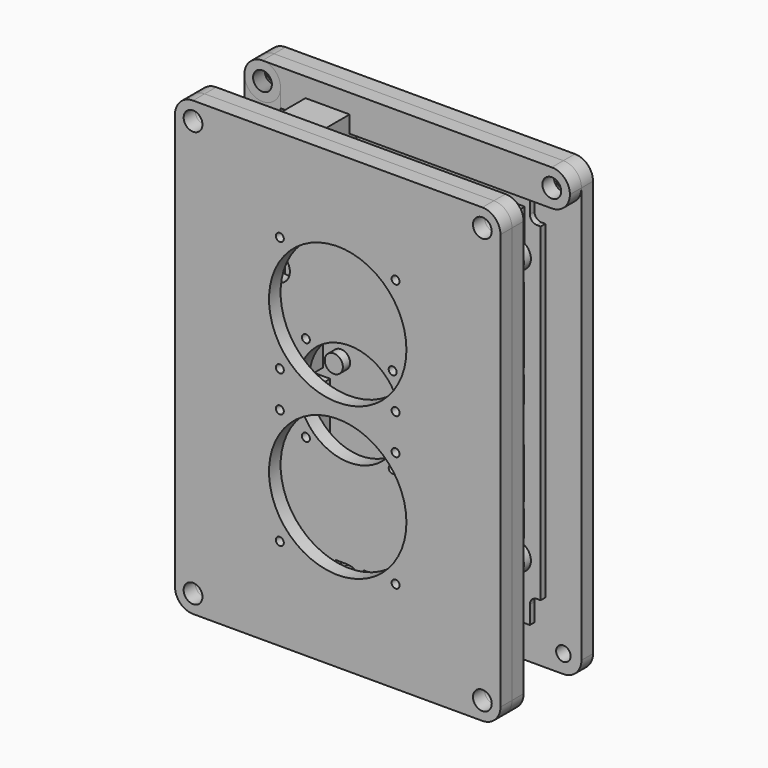
from build123d import *

# Parameters (mm, degrees)
F0_R            = 2
F0_R_2          = 1.5
F0_R_3          = 2.6
F1_DEPTH        = 4
F2_R            = 2.1
F3_DEPTH        = 4
F4_R            = 2.6
F5_DEPTH        = 4
F7_DEPTH        = 4
F8_R            = 2
F9_DEPTH        = 1.6
F10_W           = 12.2
F10_H           = 4.7
F10_H_2         = 11.8
F11_DEPTH       = 10.8
F10_W_2         = 10
F10_H_3         = 9.1
F12_DEPTH       = 12.5
F10_W_3         = 32
F10_H_4         = 7
F13_DEPTH       = 8.85
F14_SIZE2       = 4
F14_SIZE        = 1.5
F15_SIZE2       = 5
F15_SIZE        = 2
F10_W_4         = 7
F10_H_5         = 21
F16_DEPTH       = 8.8
F10_W_5         = 52.5
F10_H_6         = 9.6
F17_DEPTH       = 12.7
F10_H_7         = 14
F18_DEPTH       = 8.8
F19_SIZE2       = 4
F19_SIZE        = 1.5
F10_W_6         = 5
F10_H_8         = 7.25
F20_DEPTH       = 8.6
F21_SIZE2       = 1.5
F21_SIZE        = 4
F21_2_SIZE2     = 1.5
F21_2_SIZE      = 4
F21_3_SIZE2     = 1.5
F21_3_SIZE      = 4
F21_4_SIZE2     = 1.5
F21_4_SIZE      = 4
F21_5_SIZE2     = 1.5
F21_5_SIZE      = 4
F21_6_SIZE2     = 1.5
F21_6_SIZE      = 4
F10_R           = 2.5
F22_DEPTH       = 2.5
F23_R           = 2.6
F24_DEPTH       = 4
F26_R           = 2.6
F26_R_2         = 3.75
F27_DEPTH       = 4
F28_TEXT_SIZE   = 11.6510510219
F28_TEXT_SIZE_2 = 9.4254123618
F29_DEPTH       = 2
F30_R           = 1.1
F30_R_2         = 14.25
F31_DEPTH       = 25
F34_R           = 2.6
F34_R_2         = 1.1
F34_R_3         = 19
F35_DEPTH       = 4


# Not quite as in the source:
# - Text() gives the source's letters only with a copy of the font that has no kerning and outlines rounded to 1/6400 em; it was checked with that copy


with BuildPart() as f1:
    # F0 (on Front) → F1 (new body)
    with BuildSketch(Plane.XZ):
        with BuildLine():
            Line((-40, -62.5), (40, -62.5))
            ThreePointArc((40, -62.5), (43.5355339059, -61.0355339059), (45, -57.5))
            Line((45, -57.5), (45, 57.5))
            ThreePointArc((45, 57.5), (43.5355339059, 61.0355339059), (40, 62.5))
            Line((40, 62.5), (-40, 62.5))
            ThreePointArc((-40, 62.5), (-43.5355339059, 61.0355339059), (-45, 57.5))
            Line((-45, 57.5), (-45, -57.5))
            ThreePointArc((-45, -57.5), (-43.5355339059, -61.0355339059), (-40, -62.5))
        make_face()
        with Locations((-40, -57.5)):
            Circle(F0_R, mode=Mode.SUBTRACT)
        with Locations((-28.55, -36.75)):
            Circle(F0_R_2, mode=Mode.SUBTRACT)
        with Locations((-10, -20)):
            Circle(F0_R_3, mode=Mode.SUBTRACT)
        with Locations((40, -57.5)):
            Circle(F0_R, mode=Mode.SUBTRACT)
        with Locations((28.55, -36.75)):
            Circle(F0_R_2, mode=Mode.SUBTRACT)
        with Locations((10, -20)):
            Circle(F0_R_3, mode=Mode.SUBTRACT)
        with Locations((-10, 20)):
            Circle(F0_R_3, mode=Mode.SUBTRACT)
        with Locations((-28.55, 36.75)):
            Circle(F0_R_2, mode=Mode.SUBTRACT)
        with Locations((-40, 57.5)):
            Circle(F0_R, mode=Mode.SUBTRACT)
        with Locations((10, 20)):
            Circle(F0_R_3, mode=Mode.SUBTRACT)
        with Locations((28.55, 36.75)):
            Circle(F0_R_2, mode=Mode.SUBTRACT)
        with Locations((40, 57.5)):
            Circle(F0_R, mode=Mode.SUBTRACT)
    extrude(amount=F1_DEPTH)


with BuildPart() as f3:
    # F2 (on face) → F3 (new body)
    with BuildSketch(Plane.XZ.offset(4)):
        with BuildLine():
            ThreePointArc((-28.55, 40.5), (-32.3, 36.75), (-28.55, 33))
            Line((-28.55, 33), (28.55, 33))
            ThreePointArc((28.55, 33), (32.3, 36.75), (28.55, 40.5))
            Line((28.55, 40.5), (-28.55, 40.5))
        make_face()
        with Locations((-28.55, 36.75)):
            Circle(F2_R, mode=Mode.SUBTRACT)
        with BuildLine():
            ThreePointArc((30.65, 36.75), (28.55, 34.65), (26.45, 36.75))
            ThreePointArc((26.45, 36.75), (28.55, 38.85), (30.65, 36.75))
        make_face(mode=Mode.SUBTRACT)
    extrude(amount=F3_DEPTH)


with BuildPart() as f3b:
    # F2 (on face) → F3, piece 2 (new body)
    with BuildSketch(Plane.XZ.offset(4)):
        with BuildLine():
            ThreePointArc((-28.55, -33), (-32.3, -36.75), (-28.55, -40.5))
            Line((-28.55, -40.5), (28.55, -40.5))
            ThreePointArc((28.55, -40.5), (32.3, -36.75), (28.55, -33))
            Line((28.55, -33), (-28.55, -33))
        make_face()
        with Locations((-28.55, -36.75)):
            Circle(F2_R, mode=Mode.SUBTRACT)
        with BuildLine():
            ThreePointArc((30.65, -36.75), (28.55, -38.85), (26.45, -36.75))
            ThreePointArc((26.45, -36.75), (28.55, -34.65), (30.65, -36.75))
        make_face(mode=Mode.SUBTRACT)
    extrude(amount=F3_DEPTH)


with BuildPart() as f5:
    # F4 (on face) → F5 (new body)
    with BuildSketch(Plane.XZ.offset(4)):
        with BuildLine():
            ThreePointArc((-45, 57.5), (-43.5355339059, 53.9644660941), (-40, 52.5))
            Line((-40, 52.5), (40, 52.5))
            ThreePointArc((40, 52.5), (43.5355339059, 53.9644660941), (45, 57.5))
            ThreePointArc((45, 57.5), (43.5355339059, 61.0355339059), (40, 62.5))
            Line((40, 62.5), (-40, 62.5))
            ThreePointArc((-40, 62.5), (-43.5355339059, 61.0355339059), (-45, 57.5))
        make_face()
        with Locations((-40, 57.5)):
            Circle(F4_R, mode=Mode.SUBTRACT)
        with BuildLine():
            ThreePointArc((42.6, 57.5), (40, 54.9), (37.4, 57.5))
            ThreePointArc((37.4, 57.5), (40, 60.1), (42.6, 57.5))
        make_face(mode=Mode.SUBTRACT)
    extrude(amount=F5_DEPTH)


with BuildPart() as f7:
    # F6 (on face) → F7 (new body)
    with BuildSketch(Plane.XZ.offset(4)):
        with BuildLine():
            ThreePointArc((-40, 62.5), (-43.5355339059, 61.0355339059), (-45, 57.5))
            Line((-45, 57.5), (-45, -57.5))
            ThreePointArc((-45, -57.5), (-43.5355339059, -61.0355339059), (-40, -62.5))
            ThreePointArc((-40, -62.5), (-36.4644660941, -61.0355339059), (-35, -57.5))
            Line((-35, -57.5), (-35, 57.5))
            ThreePointArc((-35, 57.5), (-36.4644660941, 61.0355339059), (-40, 62.5))
        make_face()
        with BuildLine():
            ThreePointArc((-40, -54.9), (-38.1615223689, -55.6615223689), (-37.4, -57.5))
            ThreePointArc((-37.4, -57.5), (-41.8384776311, -59.3384776311), (-40, -54.9))
        make_face(mode=Mode.SUBTRACT)
        with BuildLine():
            ThreePointArc((-37.4, 57.5), (-38.1615223689, 55.6615223689), (-40, 54.9))
            ThreePointArc((-40, 54.9), (-41.8384776311, 59.3384776311), (-37.4, 57.5))
        make_face(mode=Mode.SUBTRACT)
    extrude(amount=F7_DEPTH)


with BuildPart() as f9:
    # F8 (on face) → F9 (new body)
    with BuildSketch(Plane.XZ.offset(4)):
        with BuildLine():
            Line((-32, -52.5), (32, -52.5))
            Line((32, -52.5), (32, -47.5))
            ThreePointArc((32, -47.5), (32.5857864376, -46.0857864376), (34, -45.5))
            Line((34, -45.5), (35, -45.5))
            Line((35, -45.5), (35, 45.5))
            Line((35, 45.5), (34, 45.5))
            ThreePointArc((34, 45.5), (32.5857864376, 46.0857864376), (32, 47.5))
            Line((32, 47.5), (32, 52.5))
            Line((32, 52.5), (-32, 52.5))
            Line((-32, 52.5), (-32, 47.5))
            ThreePointArc((-32, 47.5), (-32.5857864376, 46.0857864376), (-34, 45.5))
            Line((-34, 45.5), (-35, 45.5))
            Line((-35, 45.5), (-35, -45.5))
            Line((-35, -45.5), (-34, -45.5))
            ThreePointArc((-34, -45.5), (-32.5857864376, -46.0857864376), (-32, -47.5))
            Line((-32, -47.5), (-32, -52.5))
        make_face()
        with Locations((-28.55, -36.75)):
            Circle(F8_R, mode=Mode.SUBTRACT)
        with Locations((28.55, -36.75)):
            Circle(F8_R, mode=Mode.SUBTRACT)
        with Locations((-28.55, 36.75)):
            Circle(F8_R, mode=Mode.SUBTRACT)
        with Locations((28.55, 36.75)):
            Circle(F8_R, mode=Mode.SUBTRACT)
    extrude(amount=F9_DEPTH)


with BuildPart() as f11:
    # F10 (on face) → F11 (new body)
    with BuildSketch(Plane.XZ.offset(5.6)):
        with Locations((-22, 54.85)):
            Rectangle(F10_W, F10_H)
        with Locations((-22, 46.6)):
            Rectangle(F10_W, F10_H_2)
    extrude(amount=F11_DEPTH)


with BuildPart() as f12:
    # F10 (on face) → F12 (new body)
    with BuildSketch(Plane.XZ.offset(5.6)):
        with Locations((25.6, 44.35)):
            Rectangle(F10_W_2, F10_H_3)
    extrude(amount=F12_DEPTH)

    # F15
    f15_edges = [f12.edges().sort_by_distance(p)[0] for p in [
        (25.6, -18.1, 48.9),
    ]]
    f15_side = f12.faces().sort_by_distance((25.6, -18.1, 44.35))[0]
    chamfer(f15_edges, length=F15_SIZE, length2=F15_SIZE2, reference=f15_side)


with BuildPart() as f13:
    # F10 (on face) → F13 (new body)
    with BuildSketch(Plane.XZ.offset(5.6)):
        with Locations((2.9, 44.1)):
            Rectangle(F10_W_3, F10_H_4)
    extrude(amount=F13_DEPTH)

    # F14
    f14_edges = [f13.edges().sort_by_distance(p)[0] for p in [
        (2.9, -14.45, 47.6),
        (2.9, -14.45, 40.6),
    ]]
    f14_side = f13.faces().sort_by_distance((2.9, -14.45, 44.1))[0]
    chamfer(f14_edges, length=F14_SIZE, length2=F14_SIZE2, reference=f14_side)


with BuildPart() as f16:
    # F10 (on face) → F16 (new body)
    with BuildSketch(Plane.XZ.offset(5.6)):
        with Locations((26.85, 20)):
            Rectangle(F10_W_4, F10_H_5)
    extrude(amount=F16_DEPTH)

    # F21#3
    f21_3_edges = [f16.edges().sort_by_distance(p)[0] for p in [
        (23.35, -14.4, 20),
    ]]
    f21_3_side = f16.faces().sort_by_distance((23.35, -10, 20))[0]
    chamfer(f21_3_edges, length=F21_3_SIZE, length2=F21_3_SIZE2, reference=f21_3_side)

    # F21#4
    f21_4_edges = [f16.edges().sort_by_distance(p)[0] for p in [
        (30.35, -14.4, 20),
    ]]
    f21_4_side = f16.faces().sort_by_distance((30.35, -10, 20))[0]
    chamfer(f21_4_edges, length=F21_4_SIZE, length2=F21_4_SIZE2, reference=f21_4_side)


with BuildPart() as f16b:
    # F10 (on face) → F16, piece 2 (new body)
    with BuildSketch(Plane.XZ.offset(5.6)):
        with Locations((-26.7, 11.3)):
            Rectangle(F10_W_4, F10_H_5)
    extrude(amount=F16_DEPTH)

    # F21
    f21_edges = [f16b.edges().sort_by_distance(p)[0] for p in [
        (-30.2, -14.4, 11.3),
    ]]
    f21_side = f16b.faces().sort_by_distance((-30.2, -10, 11.3))[0]
    chamfer(f21_edges, length=F21_SIZE, length2=F21_SIZE2, reference=f21_side)

    # F21#2
    f21_2_edges = [f16b.edges().sort_by_distance(p)[0] for p in [
        (-23.2, -14.4, 11.3),
    ]]
    f21_2_side = f16b.faces().sort_by_distance((-23.2, -10, 11.3))[0]
    chamfer(f21_2_edges, length=F21_2_SIZE, length2=F21_2_SIZE2, reference=f21_2_side)


with BuildPart() as f16c:
    # F10 (on face) → F16, piece 3 (new body)
    with BuildSketch(Plane.XZ.offset(5.6)):
        with Locations((-26.7, -21)):
            Rectangle(F10_W_4, F10_H_5)
    extrude(amount=F16_DEPTH)

    # F21#5
    f21_5_edges = [f16c.edges().sort_by_distance(p)[0] for p in [
        (-30.2, -14.4, -21),
    ]]
    f21_5_side = f16c.faces().sort_by_distance((-30.2, -10, -21))[0]
    chamfer(f21_5_edges, length=F21_5_SIZE, length2=F21_5_SIZE2, reference=f21_5_side)

    # F21#6
    f21_6_edges = [f16c.edges().sort_by_distance(p)[0] for p in [
        (-23.2, -14.4, -21),
    ]]
    f21_6_side = f16c.faces().sort_by_distance((-23.2, -10, -21))[0]
    chamfer(f21_6_edges, length=F21_6_SIZE, length2=F21_6_SIZE2, reference=f21_6_side)


with BuildPart() as f17:
    # F10 (on face) → F17 (new body)
    with BuildSketch(Plane.XZ.offset(5.6)):
        with Locations((0, -46.3)):
            Rectangle(F10_W_5, F10_H_6)
    extrude(amount=F17_DEPTH)


with BuildPart() as f18:
    # F10 (on face) → F18 (new body)
    with BuildSketch(Plane.XZ.offset(5.6)):
        with Locations((26.85, -16.1)):
            Rectangle(F10_W_4, F10_H_7)
    extrude(amount=F18_DEPTH)

    # F19
    f19_edges = [f18.edges().sort_by_distance(p)[0] for p in [
        (30.35, -14.4, -16.1),
        (23.35, -14.4, -16.1),
    ]]
    f19_side = f18.faces().sort_by_distance((26.85, -14.4, -16.1))[0]
    chamfer(f19_edges, length=F19_SIZE, length2=F19_SIZE2, reference=f19_side)


with BuildPart() as f20:
    # F10 (on face) → F20 (new body)
    with BuildSketch(Plane.XZ.offset(5.6)):
        with Locations((-27.7, 27.025)):
            Rectangle(F10_W_6, F10_H_8)
    extrude(amount=F20_DEPTH)


with BuildPart() as f20b:
    # F10 (on face) → F20, piece 2 (new body)
    with BuildSketch(Plane.XZ.offset(5.6)):
        with Locations((-27.7, -4.825)):
            Rectangle(F10_W_6, F10_H_8)
    extrude(amount=F20_DEPTH)


with BuildPart() as f20c:
    # F10 (on face) → F20, piece 3 (new body)
    with BuildSketch(Plane.XZ.offset(5.6)):
        with Locations((27.85, 4.275)):
            Rectangle(F10_W_6, F10_H_8)
    extrude(amount=F20_DEPTH)


with BuildPart() as f20d:
    # F10 (on face) → F20, piece 4 (new body)
    with BuildSketch(Plane.XZ.offset(5.6)):
        with Locations((27.85, -28.325)):
            Rectangle(F10_W_6, F10_H_8)
    extrude(amount=F20_DEPTH)


with BuildPart() as f22:
    # F10 (on face) → F22 (new body)
    with BuildSketch(Plane.XZ.offset(5.6)):
        with Locations((-20.2, 27.025)):
            Circle(F10_R)
    extrude(amount=F22_DEPTH)


with BuildPart() as f22b:
    # F10 (on face) → F22, piece 2 (new body)
    with BuildSketch(Plane.XZ.offset(5.6)):
        with Locations((20.35, 4.275)):
            Circle(F10_R)
    extrude(amount=F22_DEPTH)


with BuildPart() as f22c:
    # F10 (on face) → F22, piece 3 (new body)
    with BuildSketch(Plane.XZ.offset(5.6)):
        with Locations((-20.2, -4.825)):
            Circle(F10_R)
    extrude(amount=F22_DEPTH)


with BuildPart() as f22d:
    # F10 (on face) → F22, piece 4 (new body)
    with BuildSketch(Plane.XZ.offset(5.6)):
        with Locations((20.35, -28.325)):
            Circle(F10_R)
    extrude(amount=F22_DEPTH)


with BuildPart() as f24:
    # F23 (on face) → F24 (new body)
    with BuildSketch(Plane.XZ.offset(4)):
        with BuildLine():
            ThreePointArc((-45, 57.5), (-40, 52.5), (-35, 57.5))
            ThreePointArc((-35, 57.5), (-36.4644660941, 61.0355339059), (-40, 62.5))
            ThreePointArc((-40, 62.5), (-43.5355339059, 61.0355339059), (-45, 57.5))
        make_face()
        with Locations((-40, 57.5)):
            Circle(F23_R, mode=Mode.SUBTRACT)
    extrude(amount=F24_DEPTH)


with BuildPart() as f27:
    # F26 (on offset) → F27 (new body)
    with BuildSketch(Plane.XZ.offset(24)):
        with BuildLine():
            Line((-40, -62.5), (40, -62.5))
            ThreePointArc((40, -62.5), (43.5355339059, -61.0355339059), (45, -57.5))
            Line((45, -57.5), (45, 57.5))
            ThreePointArc((45, 57.5), (43.5355339059, 61.0355339059), (40, 62.5))
            Line((40, 62.5), (-40, 62.5))
            ThreePointArc((-40, 62.5), (-43.5355339059, 61.0355339059), (-45, 57.5))
            Line((-45, 57.5), (-45, -57.5))
            ThreePointArc((-45, -57.5), (-43.5355339059, -61.0355339059), (-40, -62.5))
        make_face()
        with Locations((-40, -57.5)):
            Circle(F26_R, mode=Mode.SUBTRACT)
        with BuildLine():
            Line((-29, -31.1996527016), (-29, -10.7058370486))
            ThreePointArc((-29, -10.7058370486), (-26.5, -8.2058370486), (-24, -10.7058370486))
            Line((-24, -10.7058370486), (-24, -31.1996527016))
            ThreePointArc((-24, -31.1996527016), (-26.5, -33.6996527016), (-29, -31.1996527016))
        make_face(mode=Mode.SUBTRACT)
        with Locations((-20.2726311982, -4.8327515833)):
            Circle(F26_R_2, mode=Mode.SUBTRACT)
        with Locations((40, -57.5)):
            Circle(F26_R, mode=Mode.SUBTRACT)
        with Locations((20.3233715147, -28.3149443567)):
            Circle(F26_R_2, mode=Mode.SUBTRACT)
        with BuildLine():
            Line((24.5, -23.0461992323), (24.5, -9.053110145))
            ThreePointArc((24.5, -9.053110145), (27, -6.553110145), (29.5, -9.053110145))
            Line((29.5, -9.053110145), (29.5, -23.0461992323))
            ThreePointArc((29.5, -23.0461992323), (27, -25.5461992323), (24.5, -23.0461992323))
        make_face(mode=Mode.SUBTRACT)
        with BuildLine():
            Line((-29, 1.4001640957), (-29, 21.8920949847))
            ThreePointArc((-29, 21.8920949847), (-26.5, 24.3920949847), (-24, 21.8920949847))
            Line((-24, 21.8920949847), (-24, 1.4001640957))
            ThreePointArc((-24, 1.4001640957), (-26.5, -1.0998359043), (-29, 1.4001640957))
        make_face(mode=Mode.SUBTRACT)
        with Locations((-20.1802030206, 26.8780589104)):
            Circle(F26_R_2, mode=Mode.SUBTRACT)
        with Locations((-40, 57.5)):
            Circle(F26_R, mode=Mode.SUBTRACT)
        with Locations((20.2499870211, 4.2485971935)):
            Circle(F26_R_2, mode=Mode.SUBTRACT)
        with BuildLine():
            Line((24.5, 9.6064964309), (24.5, 30.5194072425))
            ThreePointArc((24.5, 30.5194072425), (27, 33.0194072425), (29.5, 30.5194072425))
            Line((29.5, 30.5194072425), (29.5, 9.6064964309))
            ThreePointArc((29.5, 9.6064964309), (27, 7.1064964309), (24.5, 9.6064964309))
        make_face(mode=Mode.SUBTRACT)
        with BuildLine():
            Line((30.5076725781, 41.4601838589), (-13.05074431, 41.4601838589))
            ThreePointArc((-13.05074431, 41.4601838589), (-15.55074431, 43.9601838589), (-13.05074431, 46.4601838589))
            Line((-13.05074431, 46.4601838589), (30.5076725781, 46.4601838589))
            ThreePointArc((30.5076725781, 46.4601838589), (33.0076725781, 43.9601838589), (30.5076725781, 41.4601838589))
        make_face(mode=Mode.SUBTRACT)
        with Locations((40, 57.5)):
            Circle(F26_R, mode=Mode.SUBTRACT)
    extrude(amount=F27_DEPTH)

    # F28 (on face) → F29 (cut)
    with BuildSketch(Plane.XZ.offset(28)):
        with Locations((-37.5, -47.5)):
            Text('OPENBUILDS', F28_TEXT_SIZE, font='Open Sans', font_style=FontStyle.BOLD, text_align=(TextAlign.LEFT, TextAlign.BOTTOM))
        with Locations((-32.5, 49.5820950604)):
            Text('MAKERSL.COM', F28_TEXT_SIZE_2, font='Open Sans', font_style=FontStyle.BOLDITALIC, text_align=(TextAlign.LEFT, TextAlign.BOTTOM))
    extrude(amount=-F29_DEPTH, mode=Mode.SUBTRACT)

    # F30 (on face) → F31 (cut)
    with BuildSketch(Plane.XZ.offset(28)):
        with Locations((-12, 12)):
            Circle(F30_R)
        with Locations((-12, -12)):
            Circle(F30_R)
        with Locations((12, 12)):
            Circle(F30_R)
        with Locations((12, -12)):
            Circle(F30_R)
        Circle(F30_R_2)
    extrude(amount=-F31_DEPTH, mode=Mode.SUBTRACT)


with BuildPart() as f33_1:
    # F33: copy of F27
    add(f27.part)


with BuildPart() as f35:
    # F34 (on face) → F35 (new body)
    with BuildSketch(Plane.XZ.offset(28)):
        with BuildLine():
            ThreePointArc((45, 57.5), (43.5355339059, 61.0355339059), (40, 62.5))
            Line((40, 62.5), (-40, 62.5))
            ThreePointArc((-40, 62.5), (-43.5355339059, 61.0355339059), (-45, 57.5))
            Line((-45, 57.5), (-45, -57.5))
            ThreePointArc((-45, -57.5), (-43.5355339059, -61.0355339059), (-40, -62.5))
            Line((-40, -62.5), (40, -62.5))
            ThreePointArc((40, -62.5), (43.5355339059, -61.0355339059), (45, -57.5))
            Line((45, -57.5), (45, 57.5))
        make_face()
        with Locations((-40, -57.5)):
            Circle(F34_R, mode=Mode.SUBTRACT)
        with Locations((-16, -37)):
            Circle(F34_R_2, mode=Mode.SUBTRACT)
        with Locations((-16, -5)):
            Circle(F34_R_2, mode=Mode.SUBTRACT)
        with Locations((16, -37)):
            Circle(F34_R_2, mode=Mode.SUBTRACT)
        with Locations((40, -57.5)):
            Circle(F34_R, mode=Mode.SUBTRACT)
        with Locations((0, -21)):
            Circle(F34_R_3, mode=Mode.SUBTRACT)
        with Locations((16, -5)):
            Circle(F34_R_2, mode=Mode.SUBTRACT)
        with Locations((-16, 5)):
            Circle(F34_R_2, mode=Mode.SUBTRACT)
        with Locations((-40, 57.5)):
            Circle(F34_R, mode=Mode.SUBTRACT)
        with Locations((-16, 37)):
            Circle(F34_R_2, mode=Mode.SUBTRACT)
        with Locations((16, 5)):
            Circle(F34_R_2, mode=Mode.SUBTRACT)
        with Locations((0, 21)):
            Circle(F34_R_3, mode=Mode.SUBTRACT)
        with Locations((16, 37)):
            Circle(F34_R_2, mode=Mode.SUBTRACT)
        with Locations((40, 57.5)):
            Circle(F34_R, mode=Mode.SUBTRACT)
    extrude(amount=F35_DEPTH)


solid = Compound([f1.part, f3.part, f3b.part, f5.part, f7.part, f9.part, f11.part, f12.part, f13.part, f16.part, f16b.part, f16c.part, f17.part, f18.part, f20.part, f20b.part, f20c.part, f20d.part, f22.part, f22b.part, f22c.part, f22d.part, f24.part, f27.part, f33_1.part, f35.part])
